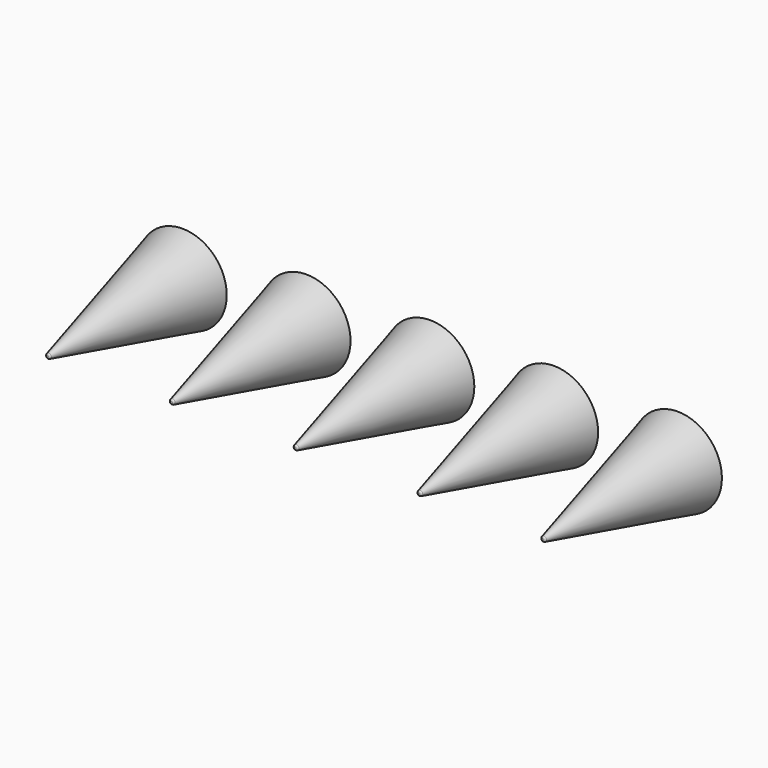
from build123d import *

# Parameters (mm, degrees)
F0_R     = 2.5
F1_DEPTH = 9.525
F1_TAPER = 14
F2_R     = 0.1
F2_2_R   = 0.1
F2_3_R   = 0.1
F2_4_R   = 0.1
F2_5_R   = 0.1


# Not quite as in the source:
# - a length typed as a fraction of an inch, garbled in the dataset ("3 / 203.2 mm" for 3/8 in), is restored


with BuildPart() as f1:
    # F0 (on Front) → F1 (new body)
    with BuildSketch(Plane.XZ):
        with Locations((-6.7453719676, 4.2574442923)):
            Circle(F0_R)
    extrude(amount=F1_DEPTH, taper=F1_TAPER)

    # F2
    f2_edges = [f1.edges().sort_by_distance(p)[0] for p in [
        (-6.870523, -9.525, 4.257444),
    ]]
    fillet(f2_edges, radius=F2_R)


with BuildPart() as f1b:
    # F0 (on Front) → F1, piece 2 (new body)
    with BuildSketch(Plane.XZ):
        with Locations((0.2546280324, 4.2574442923)):
            Circle(F0_R)
    extrude(amount=F1_DEPTH, taper=F1_TAPER)

    # F2#2
    f2_2_edges = [f1b.edges().sort_by_distance(p)[0] for p in [
        (0.129477, -9.525, 4.257444),
    ]]
    fillet(f2_2_edges, radius=F2_2_R)


with BuildPart() as f1c:
    # F0 (on Front) → F1, piece 3 (new body)
    with BuildSketch(Plane.XZ):
        with Locations((7.2546280324, 4.2574442923)):
            Circle(F0_R)
    extrude(amount=F1_DEPTH, taper=F1_TAPER)

    # F2#3
    f2_3_edges = [f1c.edges().sort_by_distance(p)[0] for p in [
        (7.129477, -9.525, 4.257444),
    ]]
    fillet(f2_3_edges, radius=F2_3_R)


with BuildPart() as f1d:
    # F0 (on Front) → F1, piece 4 (new body)
    with BuildSketch(Plane.XZ):
        with Locations((14.2546280324, 4.2574442923)):
            Circle(F0_R)
    extrude(amount=F1_DEPTH, taper=F1_TAPER)

    # F2#4
    f2_4_edges = [f1d.edges().sort_by_distance(p)[0] for p in [
        (14.129477, -9.525, 4.257444),
    ]]
    fillet(f2_4_edges, radius=F2_4_R)


with BuildPart() as f1e:
    # F0 (on Front) → F1, piece 5 (new body)
    with BuildSketch(Plane.XZ):
        with Locations((21.2546280324, 4.2574442923)):
            Circle(F0_R)
    extrude(amount=F1_DEPTH, taper=F1_TAPER)

    # F2#5
    f2_5_edges = [f1e.edges().sort_by_distance(p)[0] for p in [
        (21.129477, -9.525, 4.257444),
    ]]
    fillet(f2_5_edges, radius=F2_5_R)


solid = Compound([f1.part, f1b.part, f1c.part, f1d.part, f1e.part])
